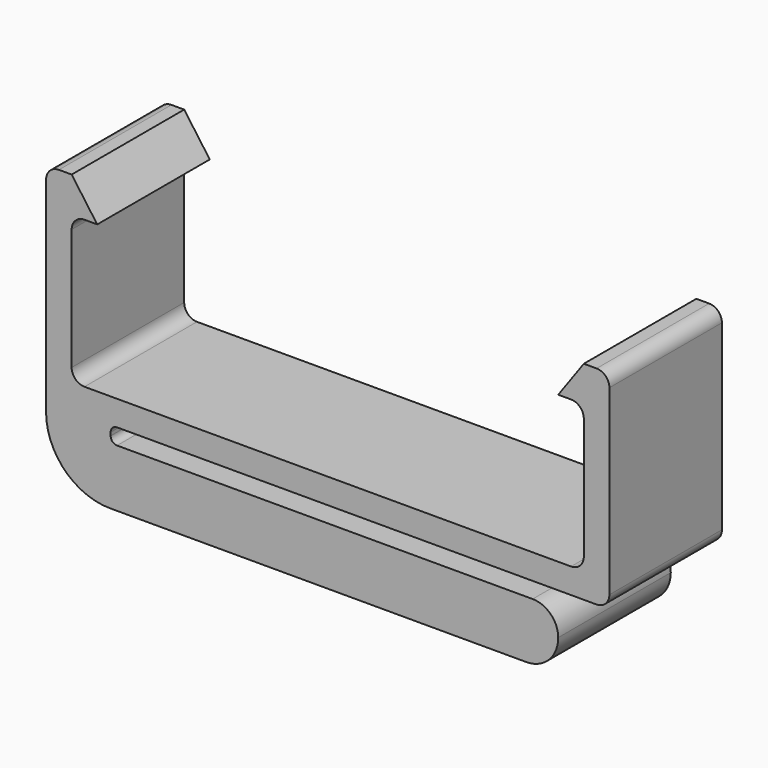
from build123d import *

# Parameters (mm, degrees)
F1_DEPTH = 22
F2_DEPTH = 5
F3_DEPTH = 5
F4_DEPTH = 5
F5_R     = 10
F6_R     = 4.99999


# Not quite as in the source:
# - a fillet or chamfer is up to 0.001 mm smaller than in the source, because OpenCascade refuses the exact size


with BuildPart() as f1:
    # F0 (on Front) → F1 (new body)
    with BuildSketch(Plane.XZ):
        with BuildLine():
            Line((-80.1, 10.8671029838), (-80.1, -15.1328970162))
            Line((-80.1, -15.1328970162), (-80.1, -21.1328970162))
            ThreePointArc((-80.1, -21.1328970162), (-78.6355339059, -24.6684309221), (-75.1, -26.1328970162))
            Line((-75.1, -26.1328970162), (0, -26.1328970162))
            ThreePointArc((0, -26.1328970162), (-1.1715728753, -23.3044698915), (-4, -22.1328970162))
            Line((-4, -22.1328970162), (-69, -22.1328970162))
            ThreePointArc((-69, -22.1328970162), (-69.7071067812, -21.8400037974), (-70, -21.1328970162))
            Line((-70, -21.1328970162), (-70, -20.6328970162))
            ThreePointArc((-70, -20.6328970162), (-69.7071067812, -19.925790235), (-69, -19.6328970162))
            Line((-69, -19.6328970162), (6, -19.6328970162))
            ThreePointArc((6, -19.6328970162), (7.4142135624, -19.0471105786), (8, -17.6328970162))
            Line((8, -17.6328970162), (8, 10.8671029838))
            ThreePointArc((8, 10.8671029838), (7.4142135624, 12.2813165462), (6, 12.8671029838))
            Line((6, 12.8671029838), (4, 12.8671029838))
            Line((4, 12.8671029838), (0, 7.3002231531))
            Line((0, 7.3002231531), (2, 7.3002231531))
            ThreePointArc((2, 7.3002231531), (3.4142135624, 6.7144367155), (4, 5.3002231531))
            Line((4, 5.3002231531), (4, -13.6997768469))
            ThreePointArc((4, -13.6997768469), (3.4142135624, -15.1139904093), (2, -15.6997768469))
            Line((2, -15.6997768469), (-74.1, -15.6997768469))
            ThreePointArc((-74.1, -15.6997768469), (-75.5142135624, -15.1139904093), (-76.1, -13.6997768469))
            Line((-76.1, -13.6997768469), (-76.1, 5.3002231531))
            ThreePointArc((-76.1, 5.3002231531), (-75.5142135624, 6.7144367155), (-74.1, 7.3002231531))
            Line((-74.1, 7.3002231531), (-72.1, 7.3002231531))
            Line((-72.1, 7.3002231531), (-76.1, 12.8671029838))
            Line((-76.1, 12.8671029838), (-78.1, 12.8671029838))
            ThreePointArc((-78.1, 12.8671029838), (-79.5142135624, 12.2813165462), (-80.1, 10.8671029838))
        make_face()
    extrude(amount=F1_DEPTH)

    # F2 (add): a face of the model
    f2_faces = [f1.faces().sort_by_distance(p)[0] for p in [
        (-37.55, -11, -26.1328970162),
    ]]
    extrude(f2_faces, amount=F2_DEPTH)

    # F3 (add, through all): a face of the model
    f3_faces = [f1.faces().sort_by_distance(p)[0] for p in [
        (-75.1, -11, -28.6328970162),
    ]]
    extrude(f3_faces, amount=F3_DEPTH)

    # F4 (add): a face of the model
    f4_faces = [f1.faces().sort_by_distance(p)[0] for p in [
        (-77.6, -11, -26.1328970162),
    ]]
    extrude(f4_faces, amount=F4_DEPTH)

    # F5
    f5_edges = [f1.edges().sort_by_distance(p)[0] for p in [
        (-80.1, -11, -31.132897),
    ]]
    fillet(f5_edges, radius=F5_R)

    # F6 (radius 5 in the source; OpenCascade refuses exactly that, so slightly less here)
    f6_edges = [f1.edges().sort_by_distance(p)[0] for p in [
        (0, -11, -31.132897),
    ]]
    fillet(f6_edges, radius=F6_R)


solid = f1.part
